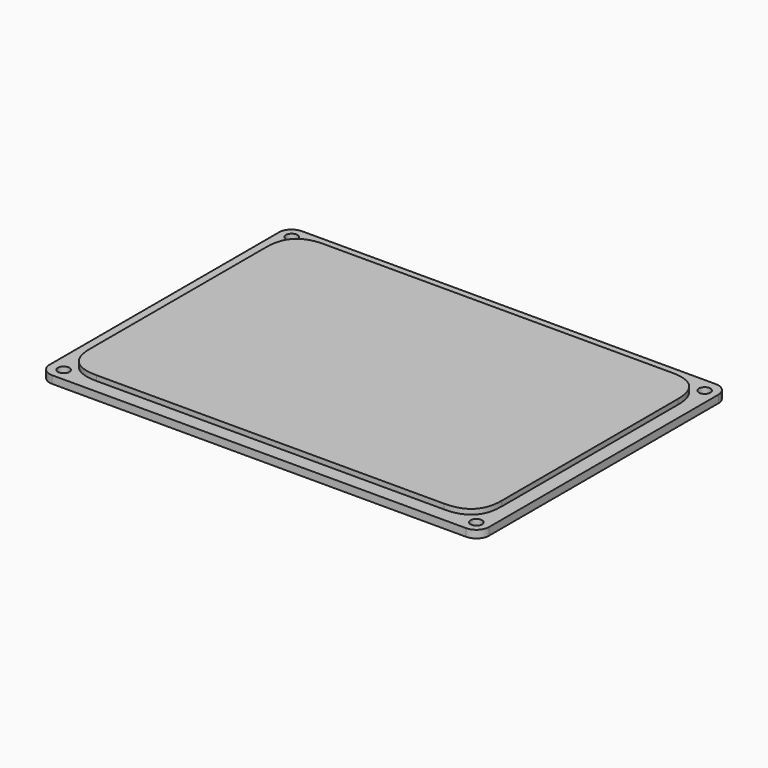
from build123d import *

# Parameters (mm, degrees)
F0_W        = 64.6
F0_H        = 44.6
F1_DEPTH    = 2
F0_W_2      = 69
F0_H_2      = 49
F2_DEPTH    = 1.2
F3_T1_DEPTH = 13.3
F4_R        = 2
F6_D        = 1.8
F6_DEPTH    = 6
F6_TIP      = 0.5407745571


# Not quite as in the source:
# - a fillet or chamfer that OpenCascade refuses, or shapes differently, is made with other operations: its cross-section is extruded or revolved along the edge and cut away or added
# - the program builds the solid bodies; features that only make, move or delete a surface that nothing else refers to are left out


with BuildPart() as f1:
    # F0 (on Top) → F1 (new body)
    with BuildSketch(Plane.XY):
        Rectangle(F0_W, F0_H)
    extrude(amount=F1_DEPTH)

    # F0 (on Top) → F2 (join)
    with BuildSketch(Plane.XY):
        Rectangle(F0_W_2, F0_H_2)
        Rectangle(F0_W, F0_H, mode=Mode.SUBTRACT)
    extrude(amount=F2_DEPTH)

    # F3: fillet of radius 5 on 4 edges, made by hand

    # F3_s2 → F3_t1 (cut)
    with BuildSketch(Plane.XY.offset(1.2)):
        with BuildLine():
            add(Edge.make_bspline(
                [(-32.3, -17.3), (-32.3, -22.3), (-27.3, -22.3)],
                knots=[0, 0, 0, 1, 1, 1], degree=2, weights=[1, 1, 1]))
            Line((-27.3, -22.3), (-32.3, -22.3))
            Line((-32.3, -22.3), (-32.3, -17.3))
        make_face()
        with BuildLine():
            add(Edge.make_bspline(
                [(32.3, -17.3), (32.3, -22.3), (27.3, -22.3)],
                knots=[0, 0, 0, 1, 1, 1], degree=2, weights=[1, 1, 1]))
            Line((27.3, -22.3), (32.3, -22.3))
            Line((32.3, -22.3), (32.3, -17.3))
        make_face()
        with BuildLine():
            add(Edge.make_bspline(
                [(27.3, 22.3), (32.3, 22.3), (32.3, 17.3)],
                knots=[0, 0, 0, 1, 1, 1], degree=2, weights=[1, 1, 1]))
            Line((32.3, 17.3), (32.3, 22.3))
            Line((32.3, 22.3), (27.3, 22.3))
        make_face()
        with BuildLine():
            add(Edge.make_bspline(
                [(-27.3, 22.3), (-32.3, 22.3), (-32.3, 17.3)],
                knots=[0, 0, 0, 1, 1, 1], degree=2, weights=[1, 1, 1]))
            Line((-32.3, 17.3), (-32.3, 22.3))
            Line((-32.3, 22.3), (-27.3, 22.3))
        make_face()
    extrude(amount=F3_T1_DEPTH, mode=Mode.SUBTRACT)

    # F4
    f4_edges = [f1.edges().sort_by_distance(p)[0] for p in [
        (-34.5, 24.5, 0.6),
        (-34.5, -24.5, 0.6),
        (34.5, 24.5, 0.6),
        (34.5, -24.5, 0.6),
    ]]
    fillet(f4_edges, radius=F4_R)

    # F6
    with Locations(Plane.XY.offset(1.2)):
        with Locations((-32.3, -22.5), (-32.5, 22.5), (32.5, -22.5), (32.5, 22.3)):
            Hole(F6_D / 2, depth=F6_DEPTH)
            with Locations((0, 0, -(F6_DEPTH + F6_TIP / 2))):  # 118° drill point
                Cone(0, F6_D / 2, F6_TIP, mode=Mode.SUBTRACT)


solid = f1.part
